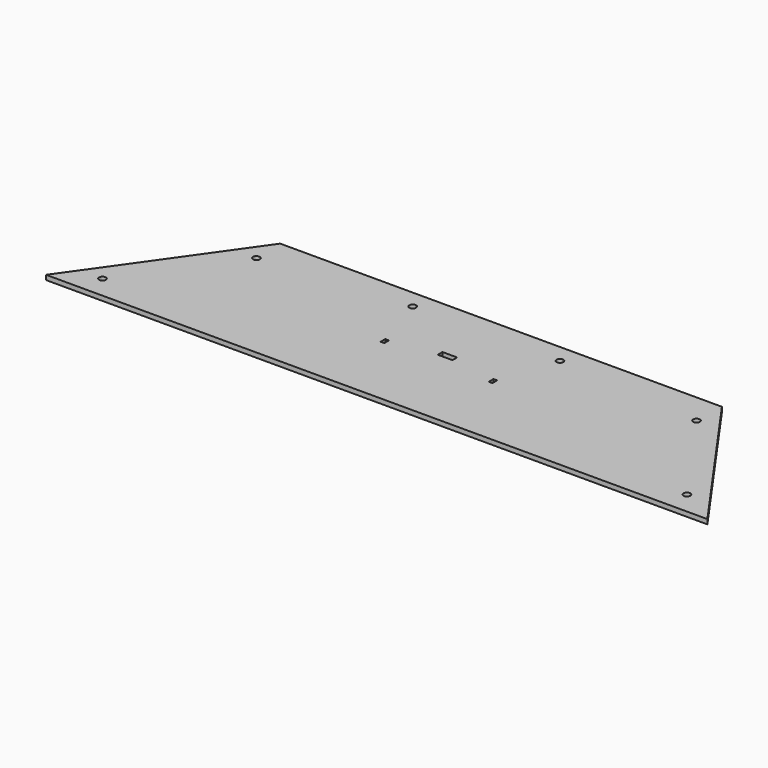
from build123d import *

# Parameters (mm, degrees)
F0_W     = 2.5
F0_H     = 4
F0_R     = 2.3114
F1_DEPTH = 3.175


with BuildPart() as f1:
    # F0 (on Top) → F1 (new body)
    with BuildSketch(Plane.XY):
        with BuildLine():
            Line((-451.5609132883, 3.4527331373), (-420.9521720122, 3.4527331373))
            Line((-420.9521720122, 3.4527331373), (-359.0199119076, 91.1230753634))
            Line((-359.0199119076, 91.1230753634), (-379.4389155629, 105.5475091382))
            Line((-379.4389155629, 105.5475091382), (-386.6511324503, 95.3380073106))
            Line((-386.6511324503, 95.3380073106), (-378.3294900246, 89.4594158723))
            ThreePointArc((-378.3294900246, 89.4594158723), (-375.7419979554, 90.3287620732), (-374.1302306227, 88.1257904232))
            ThreePointArc((-374.1302306227, 88.1257904232), (-375.3786094336, 86.0733392273), (-377.7752560717, 86.2379310212))
            Line((-377.7752560717, 86.2379310212), (-424.151080008, 20.5890373971))
            ThreePointArc((-424.151080008, 20.5890373971), (-423.4322542612, 19.7641991843), (-423.1733054571, 18.7011779952))
            ThreePointArc((-423.1733054571, 18.7011779952), (-426.1843381244, 16.4982063451), (-427.3725648591, 20.0348034442))
            Line((-427.3725648591, 20.0348034442), (-435.6942072848, 25.9133948826))
            Line((-435.6942072848, 25.9133948826), (-451.5609132883, 3.4527331373))
        make_face()
        Polygon((-359.0199119076, 91.1230753634), (-420.9521720122, 3.4527331373), (-227, 3.4527331373), (-227, 56.2263665687), (-227, 61.5263665687), (-232, 61.5263665687), (-232, 65.5263665687), (-227, 65.5263665687), (-227, 77.2140920162), (-227, 109), (-277, 109), (-377, 109), (-379.4389155629, 105.5475091382), align=None)
        with Locations((-263.75, 56.2263665687)):
            Rectangle(F0_W, F0_H, mode=Mode.SUBTRACT)
        with BuildLine():
            ThreePointArc((-274.6886, 96.5), (-278.634406614, 94.865593386), (-277, 98.8114))
            ThreePointArc((-277, 98.8114), (-275.365593386, 98.134406614), (-274.6886, 96.5))
        make_face(mode=Mode.SUBTRACT)
        Polygon((-227, 56.2263665687), (-227, 3.4527331373), (-2.4390867117, 3.4527331373), (-77, 109), (-177, 109), (-227, 109), (-227, 77.2140920162), (-227, 65.5263665687), (-222, 65.5263665687), (-222, 61.5263665687), (-227, 61.5263665687), align=None)
        with Locations((-28.5152945429, 18.7011779952)):
            Circle(F0_R, mode=Mode.SUBTRACT)
        Polygon((-191.5, 54.2263665687), (-191.5, 56.2263665687), (-191.5, 58.2263665687), (-189, 58.2263665687), (-189, 54.2263665687), align=None, mode=Mode.SUBTRACT)
        with Locations((-77.5583693773, 88.1257904232)):
            Circle(F0_R, mode=Mode.SUBTRACT)
        with BuildLine():
            ThreePointArc((-174.6886, 96.5), (-177, 94.1886), (-179.3114, 96.5))
            ThreePointArc((-179.3114, 96.5), (-178.634406614, 98.134406614), (-177, 98.8114))
            ThreePointArc((-177, 98.8114), (-175.365593386, 98.134406614), (-174.6886, 96.5))
        make_face(mode=Mode.SUBTRACT)
        with BuildLine():
            Line((-415.5, 54.5), (-435.6942072848, 25.9133948826))
            Line((-435.6942072848, 25.9133948826), (-427.3725648591, 20.0348034442))
            ThreePointArc((-427.3725648591, 20.0348034442), (-425.8766080436, 20.9791117788), (-424.151080008, 20.5890373971))
            Line((-424.151080008, 20.5890373971), (-377.7752560717, 86.2379310212))
            ThreePointArc((-377.7752560717, 86.2379310212), (-378.7195644063, 87.7338878367), (-378.3294900246, 89.4594158723))
            Line((-378.3294900246, 89.4594158723), (-386.6511324503, 95.3380073106))
            Line((-386.6511324503, 95.3380073106), (-415.5, 54.5))
        make_face()
    extrude(amount=F1_DEPTH)


solid = f1.part
